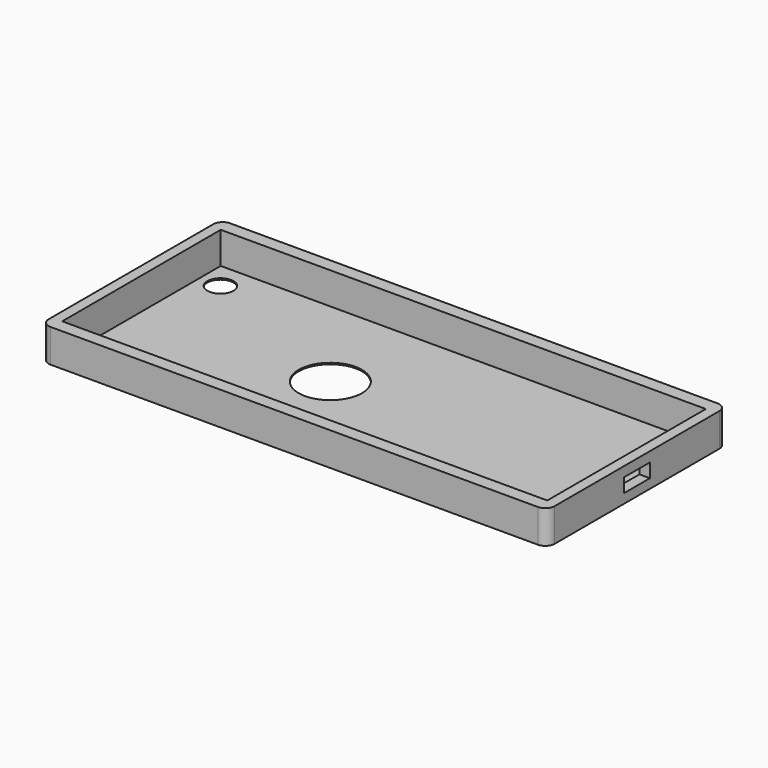
from build123d import *

# Parameters (mm, degrees)
F0_W        = 274.7335731983
F0_H        = 121.8713819981
F0_W_2      = 263.3573412895
F0_H_2      = 107.5852587819
F1_DEPTH    = 18.034
F2_W        = 263.3573412895
F2_H        = 107.5852587819
F2_R        = 7.1263998647
F2_R_2      = 17.1869969205
F3_DEPTH    = 0.762
F4_W        = 17.4885261804
F4_H        = 7.5783608481
F5_DEPTH    = 25.4
F6_W        = 17.3600167036
F6_H        = 5.2121188492
F6_W_2      = 16.0498768091
F6_H_2      = 5.5174343288
F6_W_3      = 5.82498312
F6_H_3      = 4.8827342689
F7_DEPTH    = 1.27
F8_T1_DEPTH = 22.0126396744
F8_T3_DEPTH = 22.3179551541
F8_T5_DEPTH = 21.6832550942
F9_R        = 5.08
F11_DEPTH   = 151.384


# Not quite as in the source:
# - a fillet or chamfer that OpenCascade refuses, or shapes differently, is made with other operations: its cross-section is extruded or revolved along the edge and cut away or added


with BuildPart() as f1:
    # F0 (on Top) → F1 (new body)
    with BuildSketch(Plane.XY):
        Rectangle(F0_W, F0_H)
        Rectangle(F0_W_2, F0_H_2, mode=Mode.SUBTRACT)
    extrude(amount=F1_DEPTH)

    # F4 (on face) → F5 (cut)
    with BuildSketch(Plane.YZ.offset(137.3667865992)):
        with Locations((0, 8.890000172)):
            Rectangle(F4_W, F4_H)
    extrude(amount=-F5_DEPTH, mode=Mode.SUBTRACT)

    # F6 (on face) → F7 (join)
    with BuildSketch(Plane(origin=(0, 60.935690999, 0), x_dir=(-1, 0, 0), z_dir=(0, 1, 0))):
        with Locations((55.6909367442, 11.2154921517)):
            Rectangle(F6_W, F6_H)
        with Locations((74.9413147569, 11.3532179967)):
            Rectangle(F6_W_2, F6_H_2)
        with Locations((99.9967008829, 10.7720140368)):
            Rectangle(F6_W_3, F6_H_3)
    extrude(amount=F7_DEPTH)

    # F8: fillet of radius 5.08 on 6 edges, made by hand

    # F8_s2 → F8_t1 (cut)
    with BuildSketch(Plane.XY.offset(0.2091723145)):
        with BuildLine():
            ThreePointArc((-47.0109283924, 60.935690999), (-48.5749813332, 61.8775958802), (-50.3710325575, 62.205690999))
            Line((-50.3710325575, 62.205690999), (-47.0109283924, 62.205690999))
            Line((-47.0109283924, 62.205690999), (-47.0109283924, 60.935690999))
        make_face()
        with BuildLine():
            ThreePointArc((-64.370945096, 60.935690999), (-62.8068921552, 61.8775958802), (-61.010840931, 62.205690999))
            Line((-61.010840931, 62.205690999), (-64.370945096, 62.205690999))
            Line((-64.370945096, 62.205690999), (-64.370945096, 60.935690999))
        make_face()
    extrude(amount=F8_T1_DEPTH, mode=Mode.SUBTRACT)

    # F8_s4 → F8_t3 (cut)
    with BuildSketch(Plane.XY.offset(0.1942404196)):
        with BuildLine():
            ThreePointArc((-66.9163763523, 60.935690999), (-68.4804292931, 61.8775958802), (-70.2764805174, 62.205690999))
            Line((-70.2764805174, 62.205690999), (-66.9163763523, 62.205690999))
            Line((-66.9163763523, 62.205690999), (-66.9163763523, 60.935690999))
        make_face()
        with BuildLine():
            ThreePointArc((-82.9662531614, 60.935690999), (-81.4022002206, 61.8775958802), (-79.6061489964, 62.205690999))
            Line((-79.6061489964, 62.205690999), (-82.9662531614, 62.205690999))
            Line((-82.9662531614, 62.205690999), (-82.9662531614, 60.935690999))
        make_face()
    extrude(amount=F8_T3_DEPTH, mode=Mode.SUBTRACT)

    # F8_s6 → F8_t5 (cut)
    with BuildSketch(Plane.XY.offset(-0.0696135103)):
        with BuildLine():
            ThreePointArc((-102.9091924429, 60.935690999), (-101.3451395021, 61.8775958802), (-99.5490882778, 62.205690999))
            Line((-99.5490882778, 62.205690999), (-102.9091924429, 62.205690999))
            Line((-102.9091924429, 62.205690999), (-102.9091924429, 60.935690999))
        make_face()
        with BuildLine():
            ThreePointArc((-97.0842093229, 60.935690999), (-98.6482622638, 61.8775958802), (-100.444313488, 62.205690999))
            Line((-100.444313488, 62.205690999), (-97.0842093229, 62.205690999))
            Line((-97.0842093229, 62.205690999), (-97.0842093229, 60.935690999))
        make_face()
    extrude(amount=F8_T5_DEPTH, mode=Mode.SUBTRACT)

    # F9
    f9_edges = [f1.edges().sort_by_distance(p)[0] for p in [
        (-137.366787, 60.935691, 9.017),
        (137.366787, 60.935691, 9.017),
        (137.366787, -60.935691, 9.017),
        (-137.366787, -60.935691, 9.017),
    ]]
    fillet(f9_edges, radius=F9_R)

    # F10 (on face) → F11 (cut)
    with BuildSketch(Plane(origin=(0, 0, 0), x_dir=(1, 0, 0), z_dir=(0, 0, -1))):
        with BuildLine():
            ThreePointArc((-31.5201184515, 17.0209487763), (-31.5092102693, 17.2773055673), (-31.5055732342, 17.5338685513))
            ThreePointArc((-31.5055732342, 17.5338685513), (-45.7092261373, 24.9750704372), (-43.7409795354, 9.0615150012))
            ThreePointArc((-43.7409795354, 9.0615150012), (-38.5166685327, 14.4017738694), (-31.5201184515, 17.0209487763))
        make_face()
    extrude(amount=F11_DEPTH, mode=Mode.SUBTRACT)


with BuildPart() as f3:
    # F2 (on face) → F3 (new body)
    with BuildSketch(Plane(origin=(0, 0, 0), x_dir=(1, 0, 0), z_dir=(0, 0, -1))):
        Rectangle(F2_W, F2_H)
        with Locations((-120.3147396445, -39.3977835774)):
            Circle(F2_R, mode=Mode.SUBTRACT)
        with Locations((-29.1368085891, 0)):
            Circle(F2_R_2, mode=Mode.SUBTRACT)
    extrude(amount=-F3_DEPTH)


solid = Compound([f1.part, f3.part])
